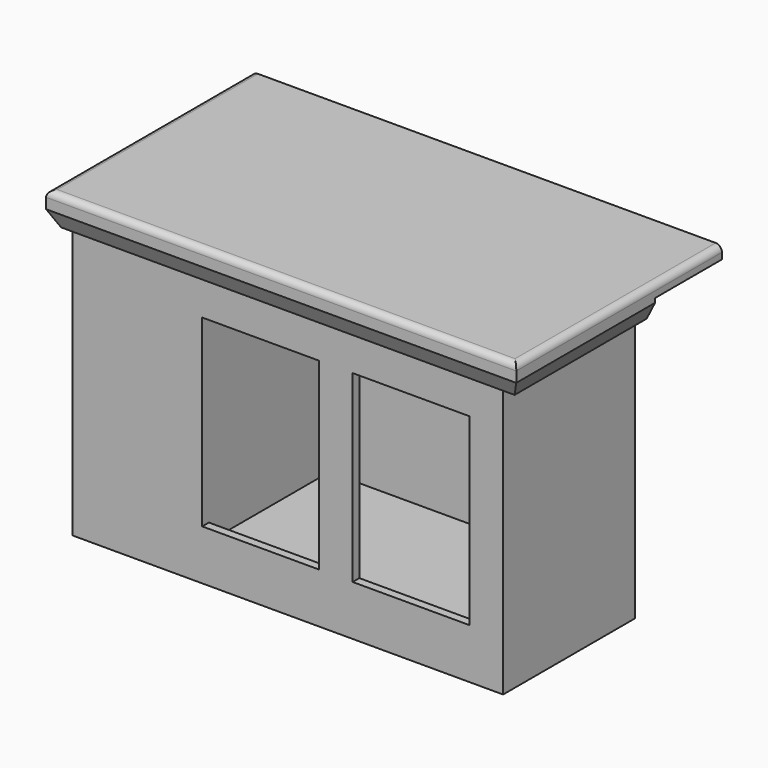
from build123d import *

# Parameters (mm, degrees)
F0_W      = 1308.1
F0_H      = 501.65
F1_DEPTH  = 812.8
F2_W      = 1428.75
F2_H      = 527.05
F3_DEPTH  = 63.5
F4_SIZE2  = 50.79999
F4_SIZE   = 25.39999
F5_W      = 1428.75
F5_H      = 527.05
F5_H_2    = 254
F6_DEPTH  = 38.1
F7_R      = 19.05
F8_W      = 355.6
F8_H      = 558.8
F9_DEPTH  = 482.6
F10_W     = 457.2
F10_H     = 558.8
F11_DEPTH = 152.4
F13_DEPTH = 50.8


# Not quite as in the source:
# - a fillet or chamfer is up to 0.001 mm smaller than in the source, because OpenCascade refuses the exact size


with BuildPart() as f1:
    # F0 (on Top) → F1 (new body)
    with BuildSketch(Plane.XY):
        with Locations((-654.05, 250.825)):
            Rectangle(F0_W, F0_H)
    extrude(amount=F1_DEPTH)

    # F2 (on face) → F3 (join)
    with BuildSketch(Plane.XY.offset(812.8)):
        with Locations((-654.05, 238.125)):
            Rectangle(F2_W, F2_H)
    extrude(amount=F3_DEPTH)

    # F4 (size 25.4 and 50.8 in the source; OpenCascade refuses exactly that, so slightly less here)
    f4_edges = [f1.edges().sort_by_distance(p)[0] for p in [
        (-1368.425, 238.125, 812.8),
        (-654.05, -25.4, 812.8),
        (60.325, 238.125, 812.8),
    ]]
    f4_side = f1.faces().sort_by_distance((-654.05, -10.171381, 812.8))[0]
    chamfer(f4_edges, length=F4_SIZE, length2=F4_SIZE2, reference=f4_side)

    # F5 (on face) → F6 (join)
    with BuildSketch(Plane.XY.offset(876.3)):
        with Locations((-654.05, 238.125)):
            Rectangle(F5_W, F5_H)
        with Locations((-654.05, 628.65)):
            Rectangle(F5_W, F5_H_2)
    extrude(amount=F6_DEPTH)

    # F7
    f7_edges = [f1.edges().sort_by_distance(p)[0] for p in [
        (-1368.425, 365.125, 914.4),
        (-654.05, -25.4, 914.4),
        (60.325, 365.125, 914.4),
    ]]
    fillet(f7_edges, radius=F7_R)

    # F8 (on face) → F9 (cut)
    with BuildSketch(Plane.XZ):
        with Locations((-279.4, 431.8)):
            Rectangle(F8_W, F8_H)
        with Locations((-736.6, 431.8)):
            Rectangle(F8_W, F8_H)
    extrude(amount=-F9_DEPTH, mode=Mode.SUBTRACT)

    # F10 (on face) → F11 (cut)
    with BuildSketch(Plane.YZ.offset(-457.2)):
        with Locations((254, 431.8)):
            Rectangle(F10_W, F10_H)
    extrude(amount=-F11_DEPTH, mode=Mode.SUBTRACT)

    # F12 (on face) → F13 (cut)
    with BuildSketch(Plane.XY.offset(152.4)):
        Polygon((-101.6, 482.6), (-914.4, 482.6), (-914.4, 25.4), (-558.8, 25.4), (-457.2, 25.4), (-101.6, 25.4), align=None)
    extrude(amount=-F13_DEPTH, mode=Mode.SUBTRACT)


solid = f1.part
